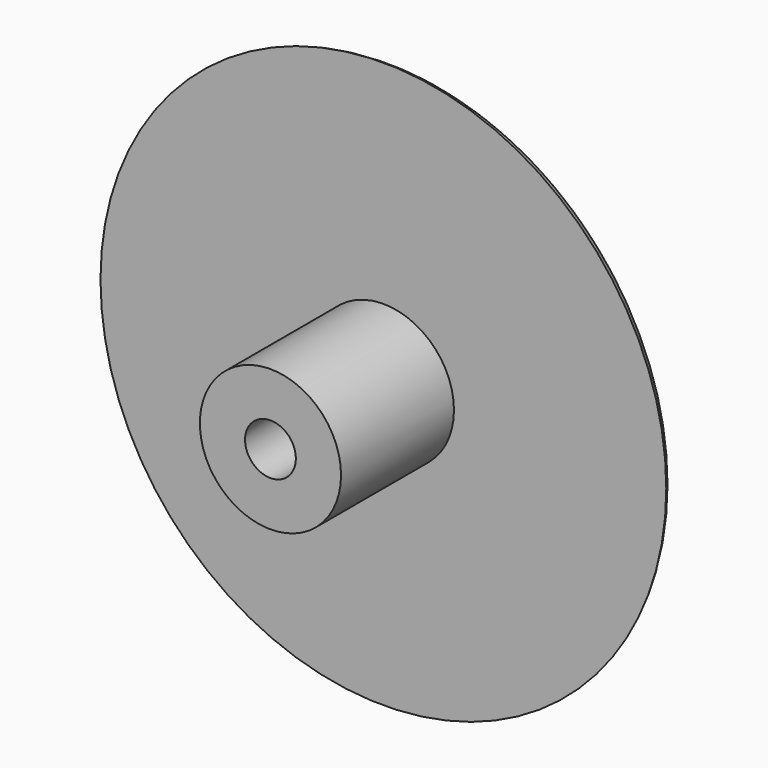
from build123d import *

# Parameters (mm, degrees)
F0_R     = 50.1
F0_R_2   = 4.5
F1_DEPTH = 3
F2_R     = 12.5
F2_R_2   = 4.5
F3_DEPTH = 25


# Not quite as in the source:
# - a fillet or chamfer that OpenCascade refuses, or shapes differently, is made with other operations: its cross-section is extruded or revolved along the edge and cut away or added


with BuildPart() as f1:
    # F0 (on Front) → F1 (new body)
    with BuildSketch(Plane.XZ):
        Circle(F0_R)
        Circle(F0_R_2, mode=Mode.SUBTRACT)
    extrude(amount=F1_DEPTH)

    # F2 (on face) → F3 (join)
    with BuildSketch(Plane.XZ.offset(3)):
        Circle(F2_R)
        Circle(F2_R_2, mode=Mode.SUBTRACT)
    extrude(amount=F3_DEPTH)

    # F4: fillet of radius 5 on 2 edges, made by hand

    # F4_s1 → F4_t2 (revolve, cut)
    with BuildSketch(Plane.XY):
        with BuildLine():
            ThreePointArc((50.1, -3), (48.2560370926, -0.8166998673), (45.517424305, 0))
            Line((45.517424305, 0), (50.1, 0))
            Line((50.1, 0), (50.1, -3))
        make_face()
    revolve(axis=Axis((0, 0, 0), (0, -1, 0)), mode=Mode.SUBTRACT)

    # F4_s3 → F4_t4 (revolve, cut)
    with BuildSketch(Plane.XY):
        with BuildLine():
            ThreePointArc((4.5, -5), (5.9644660941, -1.4644660941), (9.5, 0))
            Line((9.5, 0), (4.5, 0))
            Line((4.5, 0), (4.5, -5))
        make_face()
    revolve(axis=Axis((0, 0, 0), (0, -1, 0)), mode=Mode.SUBTRACT)


solid = f1.part
